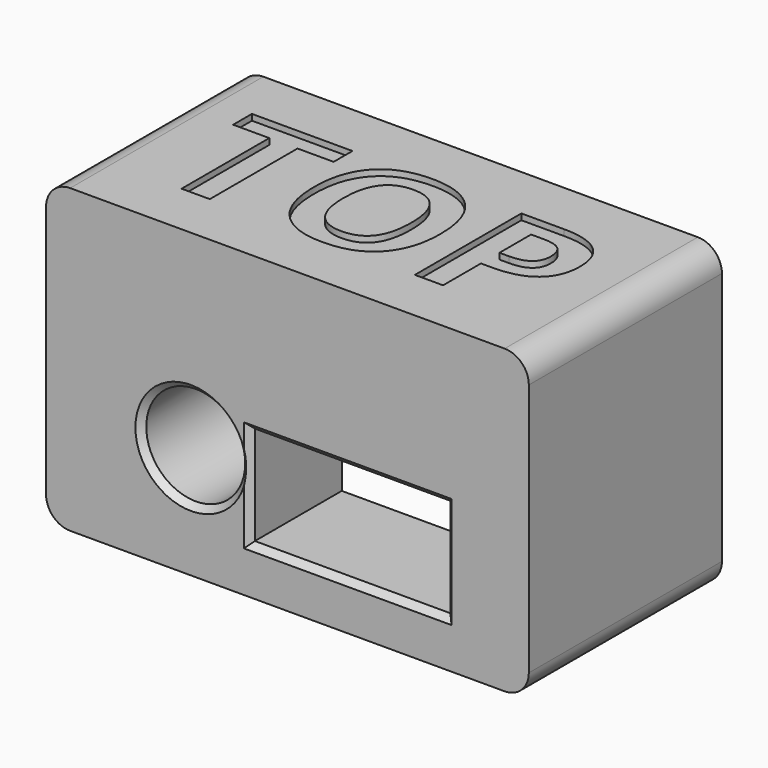
from build123d import *

# Parameters (mm, degrees)
F0_W         = 36
F0_H         = 23
F0_R         = 4.1
F0_W_2       = 16.2
F0_H_2       = 8.2
F1_DEPTH     = 10
F2_DEPTH     = 10
F3_SIZE      = 6
F4_R         = 2
F5_R         = 2
F6_TEXT_SIZE = 15.4524110258
F7_DEPTH     = 0.5
F8_T1_DEPTH  = 8.2
F8_T3_DEPTH  = 16.2
F8_T11_DEPTH = 17.485841494
F8_T15_DEPTH = 9.485841494
F8_T22_DEPTH = 9.485841494
F8_T26_DEPTH = 17.485841494
F8_T33_DEPTH = 17.485841494
F8_T37_DEPTH = 9.485841494
F8_T44_DEPTH = 17.485841494
F8_T48_DEPTH = 9.485841494
F9_T1_DEPTH  = 16.2
F9_T3_DEPTH  = 8.2
F9_T11_DEPTH = 17.485841494
F9_T15_DEPTH = 9.485841494
F9_T22_DEPTH = 17.485841494
F9_T26_DEPTH = 9.485841494
F9_T33_DEPTH = 9.485841494
F9_T37_DEPTH = 17.485841494
F9_T44_DEPTH = 17.485841494
F9_T48_DEPTH = 9.485841494


# Not quite as in the source:
# - a fillet or chamfer that OpenCascade refuses, or shapes differently, is made with other operations: its cross-section is extruded or revolved along the edge and cut away or added
# - Text() gives the source's letters only with a copy of the font that has no kerning and outlines rounded to 1/6400 em; it was checked with that copy


with BuildPart() as f1:
    # F0 (on Front) → F1 (new body)
    with BuildSketch(Plane.XZ):
        Rectangle(F0_W, F0_H)
        with Locations((-8, -2.2)):
            Circle(F0_R, mode=Mode.SUBTRACT)
        with Locations((5, -3.5)):
            Rectangle(F0_W_2, F0_H_2, mode=Mode.SUBTRACT)
        Polygon((18, 11.5), (18, -11.5), (20, -11.5), (20, 13.5), (-20, 13.5), (-20, -11.5), (-18, -11.5), (-18, 11.5), align=None)
    extrude(amount=F1_DEPTH)

    # F0 (on Front) → F2 (join)
    with BuildSketch(Plane.XZ):
        Polygon((18, 11.5), (18, -11.5), (20, -11.5), (20, 13.5), (-20, 13.5), (-20, -11.5), (-18, -11.5), (-18, 11.5), align=None)
    extrude(amount=-F2_DEPTH)

    # F3
    f3_edges = [f1.edges().sort_by_distance(p)[0] for p in [
        (-18, 5, 11.5),
    ]]
    chamfer(f3_edges, length=F3_SIZE)

    # F4
    f4_edges = [f1.edges().sort_by_distance(p)[0] for p in [
        (-20, 0, 13.5),
        (20, 0, 13.5),
    ]]
    fillet(f4_edges, radius=F4_R)

    # F5
    f5_edges = [f1.edges().sort_by_distance(p)[0] for p in [
        (20, 0, -11.5),
        (-20, 0, -11.5),
    ]]
    fillet(f5_edges, radius=F5_R)

    # F6 (on face) → F7 (cut)
    with BuildSketch(Plane.XY.offset(13.5)):
        with Locations((-15.628665089, -5.5628679693)):
            Text('TOP', F6_TEXT_SIZE, font='Open Sans', font_style=FontStyle.BOLD, text_align=(TextAlign.LEFT, TextAlign.BOTTOM))
    extrude(amount=-F7_DEPTH, mode=Mode.SUBTRACT)

    # F8: chamfer of 0.5 on 5 edges, made by hand

    # F8_s2 → F8_t1 (cut)
    with BuildSketch(Plane.XY.offset(-7.6)):
        with BuildLine():
            Line((13.6141421356, -10.0141421356), (13.0858578644, -9.4858578644))
            Line((13.0858578644, -9.4858578644), (13.0758578644, -9.4858578644))
            ThreePointArc((13.0758578644, -9.4858578644), (13.09, -9.7429289322), (13.09, -10))
            Line((13.09, -10), (13.1, -10.01))
            ThreePointArc((13.1, -10.01), (13.3570710678, -10.01), (13.6141421356, -10.0241421356))
            Line((13.6141421356, -10.0241421356), (13.6141421356, -10.0141421356))
        make_face()
        with BuildLine():
            Line((-3.6141421356, -10.0141421356), (-3.0858578644, -9.4858578644))
            Line((-3.0858578644, -9.4858578644), (-3.0758578644, -9.4858578644))
            ThreePointArc((-3.0758578644, -9.4858578644), (-3.09, -9.7429289322), (-3.09, -10))
            Line((-3.09, -10), (-3.1, -10.01))
            ThreePointArc((-3.1, -10.01), (-3.3570710678, -10.01), (-3.6141421356, -10.0241421356))
            Line((-3.6141421356, -10.0241421356), (-3.6141421356, -10.0141421356))
        make_face()
    extrude(amount=F8_T1_DEPTH, mode=Mode.SUBTRACT)

    # F8_s4 → F8_t3 (cut)
    with BuildSketch(Plane.YZ.offset(-3.1)):
        with BuildLine():
            Line((-10.0141421356, 1.1141421356), (-9.4858578644, 0.5858578644))
            Line((-9.4858578644, 0.5858578644), (-9.4858578644, 0.5758578644))
            ThreePointArc((-9.4858578644, 0.5758578644), (-9.7429289322, 0.59), (-10, 0.59))
            Line((-10, 0.59), (-10.01, 0.6))
            ThreePointArc((-10.01, 0.6), (-10.01, 0.8570710678), (-10.0241421356, 1.1141421356))
            Line((-10.0241421356, 1.1141421356), (-10.0141421356, 1.1141421356))
        make_face()
        with BuildLine():
            Line((-10.0141421356, -8.1141421356), (-9.4858578644, -7.5858578644))
            Line((-9.4858578644, -7.5858578644), (-9.4858578644, -7.5758578644))
            ThreePointArc((-9.4858578644, -7.5758578644), (-9.7429289322, -7.59), (-10, -7.59))
            Line((-10, -7.59), (-10.01, -7.6))
            ThreePointArc((-10.01, -7.6), (-10.01, -7.8570710678), (-10.0241421356, -8.1141421356))
            Line((-10.0241421356, -8.1141421356), (-10.0141421356, -8.1141421356))
        make_face()
    extrude(amount=F8_T3_DEPTH, mode=Mode.SUBTRACT)

    # F8_s5 → F8_t6 (revolve, cut)
    with BuildSketch(Plane.XY.offset(-2.2)):
        with BuildLine():
            Line((-3.3858578644, -10.0141421356), (-3.9141421356, -9.4858578644))
            Line((-3.9141421356, -9.4858578644), (-3.9241421356, -9.4858578644))
            ThreePointArc((-3.9241421356, -9.4858578644), (-3.91, -9.7429289322), (-3.91, -10))
            Line((-3.91, -10), (-3.9, -10.01))
            ThreePointArc((-3.9, -10.01), (-3.6429289322, -10.01), (-3.3858578644, -10.0241421356))
            Line((-3.3858578644, -10.0241421356), (-3.3858578644, -10.0141421356))
        make_face()
    revolve(axis=Axis((-8, -10, -2.2), (0, -1, 0)), mode=Mode.SUBTRACT)


with BuildPart() as f8_tool9:
    # F8_s10 → F8_t11 (new body)
    with BuildSketch(Plane.YZ.offset(-3.1)):
        with BuildLine():
            Line((-10.0141421356, 1.1141421356), (-9.4858578644, 0.5858578644))
            Line((-9.4858578644, 0.5858578644), (-9.4858578644, 0.5758578644))
            ThreePointArc((-9.4858578644, 0.5758578644), (-9.7429289322, 0.59), (-10, 0.59))
            Line((-10, 0.59), (-10.01, 0.6))
            ThreePointArc((-10.01, 0.6), (-10.01, 0.8570710678), (-10.0241421356, 1.1141421356))
            Line((-10.0241421356, 1.1141421356), (-10.0141421356, 1.1141421356))
        make_face()
    extrude(amount=F8_T11_DEPTH)

    split(bisect_by=Plane.YZ.offset(13.1), keep=Keep.TOP)


with BuildPart() as f8_tool13:
    # F8_s14 → F8_t15 (new body)
    with BuildSketch(Plane.XY.offset(1.885841494)):
        with BuildLine():
            Line((13.6141421356, -10.0141421356), (13.0858578644, -9.4858578644))
            Line((13.0858578644, -9.4858578644), (13.0758578644, -9.4858578644))
            ThreePointArc((13.0758578644, -9.4858578644), (13.09, -9.7429289322), (13.09, -10))
            Line((13.09, -10), (13.1, -10.01))
            ThreePointArc((13.1, -10.01), (13.3570710678, -10.01), (13.6141421356, -10.0241421356))
            Line((13.6141421356, -10.0241421356), (13.6141421356, -10.0141421356))
        make_face()
    extrude(amount=-F8_T15_DEPTH)

    split(bisect_by=Plane.XY.offset(0.6), keep=Keep.TOP)


with BuildPart() as f8_tool9_1:
    add(f8_tool9.part)

    # F8_t17: intersect F8_tool13
    add(f8_tool13.part, mode=Mode.INTERSECT)


with BuildPart() as f1_1:
    add(f1.part)

    # F8_t7: cut F8_tool9
    add(f8_tool9_1.part, mode=Mode.SUBTRACT)


with BuildPart() as f8_tool20:
    # F8_s21 → F8_t22 (new body)
    with BuildSketch(Plane.XY.offset(0.6)):
        with BuildLine():
            Line((13.6141421356, -10.0141421356), (13.0858578644, -9.4858578644))
            Line((13.0858578644, -9.4858578644), (13.0758578644, -9.4858578644))
            ThreePointArc((13.0758578644, -9.4858578644), (13.09, -9.7429289322), (13.09, -10))
            Line((13.09, -10), (13.1, -10.01))
            ThreePointArc((13.1, -10.01), (13.3570710678, -10.01), (13.6141421356, -10.0241421356))
            Line((13.6141421356, -10.0241421356), (13.6141421356, -10.0141421356))
        make_face()
    extrude(amount=-F8_T22_DEPTH)

    split(bisect_by=Plane.XY.offset(-7.6), keep=Keep.BOTTOM)


with BuildPart() as f8_tool24:
    # F8_s25 → F8_t26 (new body)
    with BuildSketch(Plane.YZ.offset(14.385841494)):
        with BuildLine():
            Line((-10.0141421356, -8.1141421356), (-9.4858578644, -7.5858578644))
            Line((-9.4858578644, -7.5858578644), (-9.4858578644, -7.5758578644))
            ThreePointArc((-9.4858578644, -7.5758578644), (-9.7429289322, -7.59), (-10, -7.59))
            Line((-10, -7.59), (-10.01, -7.6))
            ThreePointArc((-10.01, -7.6), (-10.01, -7.8570710678), (-10.0241421356, -8.1141421356))
            Line((-10.0241421356, -8.1141421356), (-10.0141421356, -8.1141421356))
        make_face()
    extrude(amount=-F8_T26_DEPTH)

    split(bisect_by=Plane.YZ.offset(13.1), keep=Keep.TOP)


with BuildPart() as f8_tool20_1:
    add(f8_tool20.part)

    # F8_t28: intersect F8_tool24
    add(f8_tool24.part, mode=Mode.INTERSECT)


with BuildPart() as f1_2:
    add(f1_1.part)

    # F8_t18: cut F8_tool20
    add(f8_tool20_1.part, mode=Mode.SUBTRACT)


with BuildPart() as f8_tool31:
    # F8_s32 → F8_t33 (new body)
    with BuildSketch(Plane.YZ.offset(-4.385841494)):
        with BuildLine():
            Line((-10.0141421356, 1.1141421356), (-9.4858578644, 0.5858578644))
            Line((-9.4858578644, 0.5858578644), (-9.4858578644, 0.5758578644))
            ThreePointArc((-9.4858578644, 0.5758578644), (-9.7429289322, 0.59), (-10, 0.59))
            Line((-10, 0.59), (-10.01, 0.6))
            ThreePointArc((-10.01, 0.6), (-10.01, 0.8570710678), (-10.0241421356, 1.1141421356))
            Line((-10.0241421356, 1.1141421356), (-10.0141421356, 1.1141421356))
        make_face()
    extrude(amount=F8_T33_DEPTH)

    split(bisect_by=Plane.YZ.offset(-3.1), keep=Keep.BOTTOM)


with BuildPart() as f8_tool35:
    # F8_s36 → F8_t37 (new body)
    with BuildSketch(Plane.XY.offset(-7.6)):
        with BuildLine():
            Line((-3.6141421356, -10.0141421356), (-3.0858578644, -9.4858578644))
            Line((-3.0858578644, -9.4858578644), (-3.0758578644, -9.4858578644))
            ThreePointArc((-3.0758578644, -9.4858578644), (-3.09, -9.7429289322), (-3.09, -10))
            Line((-3.09, -10), (-3.1, -10.01))
            ThreePointArc((-3.1, -10.01), (-3.3570710678, -10.01), (-3.6141421356, -10.0241421356))
            Line((-3.6141421356, -10.0241421356), (-3.6141421356, -10.0141421356))
        make_face()
    extrude(amount=F8_T37_DEPTH)

    split(bisect_by=Plane.XY.offset(0.6), keep=Keep.TOP)


with BuildPart() as f8_tool31_1:
    add(f8_tool31.part)

    # F8_t39: intersect F8_tool35
    add(f8_tool35.part, mode=Mode.INTERSECT)


with BuildPart() as f1_3:
    add(f1_2.part)

    # F8_t29: cut F8_tool31
    add(f8_tool31_1.part, mode=Mode.SUBTRACT)


with BuildPart() as f8_tool42:
    # F8_s43 → F8_t44 (new body)
    with BuildSketch(Plane.YZ.offset(13.1)):
        with BuildLine():
            Line((-10.0141421356, -8.1141421356), (-9.4858578644, -7.5858578644))
            Line((-9.4858578644, -7.5858578644), (-9.4858578644, -7.5758578644))
            ThreePointArc((-9.4858578644, -7.5758578644), (-9.7429289322, -7.59), (-10, -7.59))
            Line((-10, -7.59), (-10.01, -7.6))
            ThreePointArc((-10.01, -7.6), (-10.01, -7.8570710678), (-10.0241421356, -8.1141421356))
            Line((-10.0241421356, -8.1141421356), (-10.0141421356, -8.1141421356))
        make_face()
    extrude(amount=-F8_T44_DEPTH)

    split(bisect_by=Plane.YZ.offset(-3.1), keep=Keep.BOTTOM)


with BuildPart() as f8_tool46:
    # F8_s47 → F8_t48 (new body)
    with BuildSketch(Plane.XY.offset(-8.885841494)):
        with BuildLine():
            Line((-3.6141421356, -10.0141421356), (-3.0858578644, -9.4858578644))
            Line((-3.0858578644, -9.4858578644), (-3.0758578644, -9.4858578644))
            ThreePointArc((-3.0758578644, -9.4858578644), (-3.09, -9.7429289322), (-3.09, -10))
            Line((-3.09, -10), (-3.1, -10.01))
            ThreePointArc((-3.1, -10.01), (-3.3570710678, -10.01), (-3.6141421356, -10.0241421356))
            Line((-3.6141421356, -10.0241421356), (-3.6141421356, -10.0141421356))
        make_face()
    extrude(amount=F8_T48_DEPTH)

    split(bisect_by=Plane.XY.offset(-7.6), keep=Keep.BOTTOM)


with BuildPart() as f8_tool42_1:
    add(f8_tool42.part)

    # F8_t50: intersect F8_tool46
    add(f8_tool46.part, mode=Mode.INTERSECT)


with BuildPart() as f1_4:
    add(f1_3.part)

    # F8_t40: cut F8_tool42
    add(f8_tool42_1.part, mode=Mode.SUBTRACT)

    # F9: chamfer of 0.5 on 5 edges, made by hand

    # F9_s2 → F9_t1 (cut)
    with BuildSketch(Plane.YZ.offset(-3.1)):
        with BuildLine():
            Line((-0.5141421356, -7.5858578644), (0.0141421356, -8.1141421356))
            Line((0.0141421356, -8.1141421356), (0.0241421356, -8.1141421356))
            ThreePointArc((0.0241421356, -8.1141421356), (0.01, -7.8570710678), (0.01, -7.6))
            Line((0.01, -7.6), (0, -7.59))
            ThreePointArc((0, -7.59), (-0.2570710678, -7.59), (-0.5141421356, -7.5758578644))
            Line((-0.5141421356, -7.5758578644), (-0.5141421356, -7.5858578644))
        make_face()
        with BuildLine():
            Line((-0.5141421356, 0.5858578644), (0.0141421356, 1.1141421356))
            Line((0.0141421356, 1.1141421356), (0.0241421356, 1.1141421356))
            ThreePointArc((0.0241421356, 1.1141421356), (0.01, 0.8570710678), (0.01, 0.6))
            Line((0.01, 0.6), (0, 0.59))
            ThreePointArc((0, 0.59), (-0.2570710678, 0.59), (-0.5141421356, 0.5758578644))
            Line((-0.5141421356, 0.5758578644), (-0.5141421356, 0.5858578644))
        make_face()
    extrude(amount=F9_T1_DEPTH, mode=Mode.SUBTRACT)

    # F9_s4 → F9_t3 (cut)
    with BuildSketch(Plane.XY.offset(-7.6)):
        with BuildLine():
            Line((-3.0858578644, -0.5141421356), (-3.6141421356, 0.0141421356))
            Line((-3.6141421356, 0.0141421356), (-3.6141421356, 0.0241421356))
            ThreePointArc((-3.6141421356, 0.0241421356), (-3.3570710678, 0.01), (-3.1, 0.01))
            Line((-3.1, 0.01), (-3.09, 0))
            ThreePointArc((-3.09, 0), (-3.09, -0.2570710678), (-3.0758578644, -0.5141421356))
            Line((-3.0758578644, -0.5141421356), (-3.0858578644, -0.5141421356))
        make_face()
        with BuildLine():
            Line((13.6141421356, 0.0141421356), (13.0858578644, -0.5141421356))
            Line((13.0858578644, -0.5141421356), (13.0758578644, -0.5141421356))
            ThreePointArc((13.0758578644, -0.5141421356), (13.09, -0.2570710678), (13.09, 0))
            Line((13.09, 0), (13.1, 0.01))
            ThreePointArc((13.1, 0.01), (13.3570710678, 0.01), (13.6141421356, 0.0241421356))
            Line((13.6141421356, 0.0241421356), (13.6141421356, 0.0141421356))
        make_face()
    extrude(amount=F9_T3_DEPTH, mode=Mode.SUBTRACT)

    # F9_s5 → F9_t6 (revolve, cut)
    with BuildSketch(Plane.XY.offset(-2.2)):
        with BuildLine():
            Line((-3.3858578644, 0.0141421356), (-3.9141421356, -0.5141421356))
            Line((-3.9141421356, -0.5141421356), (-3.9241421356, -0.5141421356))
            ThreePointArc((-3.9241421356, -0.5141421356), (-3.91, -0.2570710678), (-3.91, 0))
            Line((-3.91, 0), (-3.9, 0.01))
            ThreePointArc((-3.9, 0.01), (-3.6429289322, 0.01), (-3.3858578644, 0.0241421356))
            Line((-3.3858578644, 0.0241421356), (-3.3858578644, 0.0141421356))
        make_face()
    revolve(axis=Axis((-8, 0, -2.2), (0, -1, 0)), mode=Mode.SUBTRACT)


with BuildPart() as f9_tool9:
    # F9_s10 → F9_t11 (new body)
    with BuildSketch(Plane.YZ.offset(14.385841494)):
        with BuildLine():
            Line((-0.5141421356, -7.5858578644), (0.0141421356, -8.1141421356))
            Line((0.0141421356, -8.1141421356), (0.0241421356, -8.1141421356))
            ThreePointArc((0.0241421356, -8.1141421356), (0.01, -7.8570710678), (0.01, -7.6))
            Line((0.01, -7.6), (0, -7.59))
            ThreePointArc((0, -7.59), (-0.2570710678, -7.59), (-0.5141421356, -7.5758578644))
            Line((-0.5141421356, -7.5758578644), (-0.5141421356, -7.5858578644))
        make_face()
    extrude(amount=-F9_T11_DEPTH)

    split(bisect_by=Plane.YZ.offset(13.1), keep=Keep.TOP)


with BuildPart() as f9_tool13:
    # F9_s14 → F9_t15 (new body)
    with BuildSketch(Plane.XY.offset(0.6)):
        with BuildLine():
            Line((13.6141421356, 0.0141421356), (13.0858578644, -0.5141421356))
            Line((13.0858578644, -0.5141421356), (13.0758578644, -0.5141421356))
            ThreePointArc((13.0758578644, -0.5141421356), (13.09, -0.2570710678), (13.09, 0))
            Line((13.09, 0), (13.1, 0.01))
            ThreePointArc((13.1, 0.01), (13.3570710678, 0.01), (13.6141421356, 0.0241421356))
            Line((13.6141421356, 0.0241421356), (13.6141421356, 0.0141421356))
        make_face()
    extrude(amount=-F9_T15_DEPTH)

    split(bisect_by=Plane.XY.offset(-7.6), keep=Keep.BOTTOM)


with BuildPart() as f9_tool9_1:
    add(f9_tool9.part)

    # F9_t17: intersect F9_tool13
    add(f9_tool13.part, mode=Mode.INTERSECT)


with BuildPart() as f1_5:
    add(f1_4.part)

    # F9_t7: cut F9_tool9
    add(f9_tool9_1.part, mode=Mode.SUBTRACT)


with BuildPart() as f9_tool20:
    # F9_s21 → F9_t22 (new body)
    with BuildSketch(Plane.YZ.offset(13.1)):
        with BuildLine():
            Line((-0.5141421356, -7.5858578644), (0.0141421356, -8.1141421356))
            Line((0.0141421356, -8.1141421356), (0.0241421356, -8.1141421356))
            ThreePointArc((0.0241421356, -8.1141421356), (0.01, -7.8570710678), (0.01, -7.6))
            Line((0.01, -7.6), (0, -7.59))
            ThreePointArc((0, -7.59), (-0.2570710678, -7.59), (-0.5141421356, -7.5758578644))
            Line((-0.5141421356, -7.5758578644), (-0.5141421356, -7.5858578644))
        make_face()
    extrude(amount=-F9_T22_DEPTH)

    split(bisect_by=Plane.YZ.offset(-3.1), keep=Keep.BOTTOM)


with BuildPart() as f9_tool24:
    # F9_s25 → F9_t26 (new body)
    with BuildSketch(Plane.XY.offset(-8.885841494)):
        with BuildLine():
            Line((-3.0858578644, -0.5141421356), (-3.6141421356, 0.0141421356))
            Line((-3.6141421356, 0.0141421356), (-3.6141421356, 0.0241421356))
            ThreePointArc((-3.6141421356, 0.0241421356), (-3.3570710678, 0.01), (-3.1, 0.01))
            Line((-3.1, 0.01), (-3.09, 0))
            ThreePointArc((-3.09, 0), (-3.09, -0.2570710678), (-3.0758578644, -0.5141421356))
            Line((-3.0758578644, -0.5141421356), (-3.0858578644, -0.5141421356))
        make_face()
    extrude(amount=F9_T26_DEPTH)

    split(bisect_by=Plane.XY.offset(-7.6), keep=Keep.BOTTOM)


with BuildPart() as f9_tool20_1:
    add(f9_tool20.part)

    # F9_t28: intersect F9_tool24
    add(f9_tool24.part, mode=Mode.INTERSECT)


with BuildPart() as f1_6:
    add(f1_5.part)

    # F9_t18: cut F9_tool20
    add(f9_tool20_1.part, mode=Mode.SUBTRACT)


with BuildPart() as f9_tool31:
    # F9_s32 → F9_t33 (new body)
    with BuildSketch(Plane.XY.offset(-7.6)):
        with BuildLine():
            Line((-3.0858578644, -0.5141421356), (-3.6141421356, 0.0141421356))
            Line((-3.6141421356, 0.0141421356), (-3.6141421356, 0.0241421356))
            ThreePointArc((-3.6141421356, 0.0241421356), (-3.3570710678, 0.01), (-3.1, 0.01))
            Line((-3.1, 0.01), (-3.09, 0))
            ThreePointArc((-3.09, 0), (-3.09, -0.2570710678), (-3.0758578644, -0.5141421356))
            Line((-3.0758578644, -0.5141421356), (-3.0858578644, -0.5141421356))
        make_face()
    extrude(amount=F9_T33_DEPTH)

    split(bisect_by=Plane.XY.offset(0.6), keep=Keep.TOP)


with BuildPart() as f9_tool35:
    # F9_s36 → F9_t37 (new body)
    with BuildSketch(Plane.YZ.offset(-4.385841494)):
        with BuildLine():
            Line((-0.5141421356, 0.5858578644), (0.0141421356, 1.1141421356))
            Line((0.0141421356, 1.1141421356), (0.0241421356, 1.1141421356))
            ThreePointArc((0.0241421356, 1.1141421356), (0.01, 0.8570710678), (0.01, 0.6))
            Line((0.01, 0.6), (0, 0.59))
            ThreePointArc((0, 0.59), (-0.2570710678, 0.59), (-0.5141421356, 0.5758578644))
            Line((-0.5141421356, 0.5758578644), (-0.5141421356, 0.5858578644))
        make_face()
    extrude(amount=F9_T37_DEPTH)

    split(bisect_by=Plane.YZ.offset(-3.1), keep=Keep.BOTTOM)


with BuildPart() as f9_tool31_1:
    add(f9_tool31.part)

    # F9_t39: intersect F9_tool35
    add(f9_tool35.part, mode=Mode.INTERSECT)


with BuildPart() as f1_7:
    add(f1_6.part)

    # F9_t29: cut F9_tool31
    add(f9_tool31_1.part, mode=Mode.SUBTRACT)


with BuildPart() as f9_tool42:
    # F9_s43 → F9_t44 (new body)
    with BuildSketch(Plane.YZ.offset(-3.1)):
        with BuildLine():
            Line((-0.5141421356, 0.5858578644), (0.0141421356, 1.1141421356))
            Line((0.0141421356, 1.1141421356), (0.0241421356, 1.1141421356))
            ThreePointArc((0.0241421356, 1.1141421356), (0.01, 0.8570710678), (0.01, 0.6))
            Line((0.01, 0.6), (0, 0.59))
            ThreePointArc((0, 0.59), (-0.2570710678, 0.59), (-0.5141421356, 0.5758578644))
            Line((-0.5141421356, 0.5758578644), (-0.5141421356, 0.5858578644))
        make_face()
    extrude(amount=F9_T44_DEPTH)

    split(bisect_by=Plane.YZ.offset(13.1), keep=Keep.TOP)


with BuildPart() as f9_tool46:
    # F9_s47 → F9_t48 (new body)
    with BuildSketch(Plane.XY.offset(1.885841494)):
        with BuildLine():
            Line((13.6141421356, 0.0141421356), (13.0858578644, -0.5141421356))
            Line((13.0858578644, -0.5141421356), (13.0758578644, -0.5141421356))
            ThreePointArc((13.0758578644, -0.5141421356), (13.09, -0.2570710678), (13.09, 0))
            Line((13.09, 0), (13.1, 0.01))
            ThreePointArc((13.1, 0.01), (13.3570710678, 0.01), (13.6141421356, 0.0241421356))
            Line((13.6141421356, 0.0241421356), (13.6141421356, 0.0141421356))
        make_face()
    extrude(amount=-F9_T48_DEPTH)

    split(bisect_by=Plane.XY.offset(0.6), keep=Keep.TOP)


with BuildPart() as f9_tool42_1:
    add(f9_tool42.part)

    # F9_t50: intersect F9_tool46
    add(f9_tool46.part, mode=Mode.INTERSECT)


with BuildPart() as f1_8:
    add(f1_7.part)

    # F9_t40: cut F9_tool42
    add(f9_tool42_1.part, mode=Mode.SUBTRACT)


solid = f1_8.part
